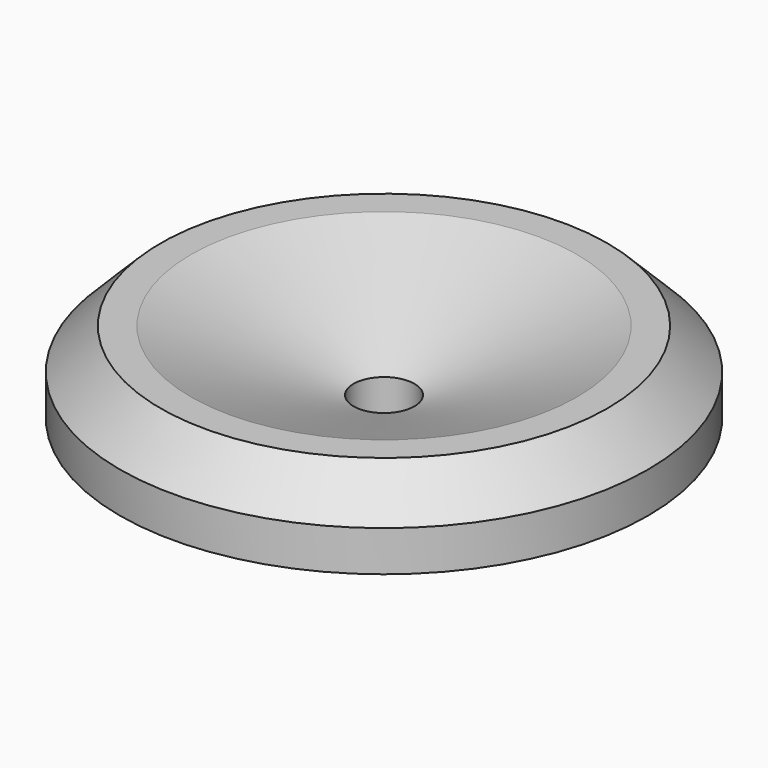
from build123d import *

# Parameters (mm, degrees)
F0_R     = 13
F1_DEPTH = 4
F2_SIZE  = 2
F3_R     = 4.7
F4_DEPTH = 3.5
F5_SIZE  = 0.5
F6_R     = 1.5
F7_DEPTH = 25
F8_R     = 5.7
F8_R_2   = 4.7
F9_DEPTH = 1.5


# Not quite as in the source:
# - a fillet or chamfer that OpenCascade refuses, or shapes differently, is made with other operations: its cross-section is extruded or revolved along the edge and cut away or added


with BuildPart() as f1:
    # F0 (on Top) → F1 (new body)
    with BuildSketch(Plane.XY):
        Circle(F0_R)
    extrude(amount=F1_DEPTH)

    # F2
    f2_edges = [f1.edges().sort_by_distance(p)[0] for p in [
        (-13, 0, 4),
    ]]
    chamfer(f2_edges, length=F2_SIZE)

    # F3 (on face) → F4 (join)
    with BuildSketch(Plane(origin=(0, 0, 0), x_dir=(1, 0, 0), z_dir=(0, 0, -1))):
        Circle(F3_R)
    extrude(amount=F4_DEPTH)

    # F5
    f5_edges = [f1.edges().sort_by_distance(p)[0] for p in [
        (-4.7, 0, -3.5),
    ]]
    chamfer(f5_edges, length=F5_SIZE)

    # F6 (on face) → F7 (cut)
    with BuildSketch(Plane(origin=(0, 0, -3.5), x_dir=(1, 0, 0), z_dir=(0, 0, -1))):
        Circle(F6_R)
    extrude(amount=-F7_DEPTH, mode=Mode.SUBTRACT)

    # F8 (on face) → F9 (join)
    with BuildSketch(Plane(origin=(0, 0, 0), x_dir=(1, 0, 0), z_dir=(0, 0, -1))):
        Circle(F8_R)
        Circle(F8_R_2, mode=Mode.SUBTRACT)
    extrude(amount=F9_DEPTH)

    # F10: chamfer of 3 x 8 on 1 edges, made by hand

    # F10_s1 → F10_t2 (revolve, cut)
    with BuildSketch(Plane.XZ):
        Polygon((1.5, 1), (9.5, 4), (1.5, 4), align=None)
    revolve(axis=Axis((0, 0, 4), (0, 0, -1)), mode=Mode.SUBTRACT)


solid = f1.part
